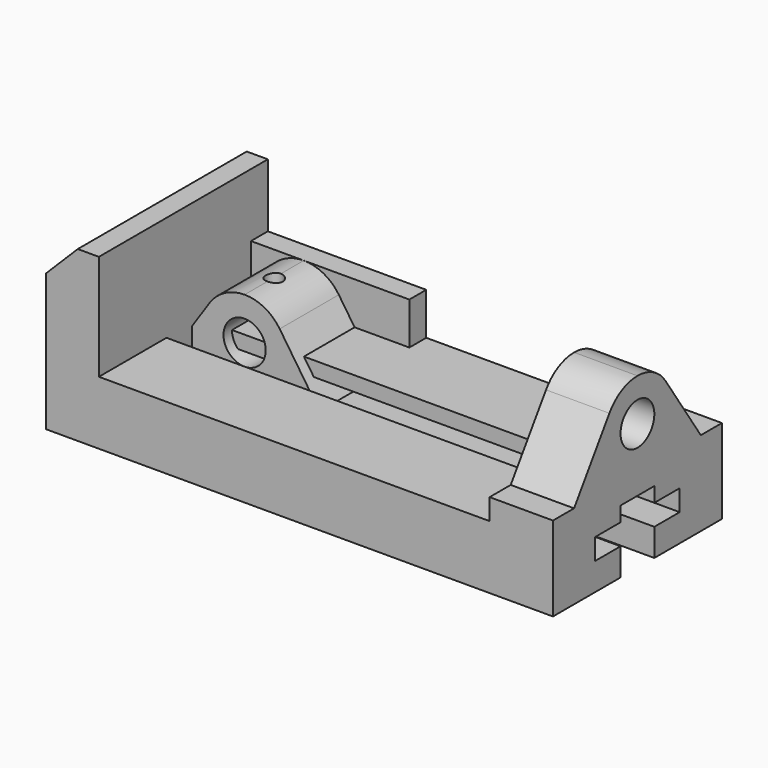
from build123d import *

# Parameters (mm, degrees)
F1_DEPTH  = 127
F2_SIZE2  = 19.05
F2_SIZE   = 19.05
F4_DEPTH  = 273.05
F5_R      = 12.7
F6_DEPTH  = 38.101
F8_DEPTH  = 57.15
F10_DEPTH = 44.45
F9_R      = 12.7
F11_DEPTH = 57.151
F12_R     = 5.08
F13_REACH = 99.4594097937
F14_R     = 12.7
F15_DEPTH = 279.4
F17_DEPTH = 25.4
F18_DEPTH = 2.54
F19_R     = 4.445
F20_DEPTH = 76.2


with BuildPart() as f1:
    # F0 (on Front) → F1 (new body)
    with BuildSketch(Plane.XZ):
        Polygon((31.75, 38.1), (31.75, 101.6), (0, 101.6), (0, 0), (304.8, 0), (304.8, 101.6), (266.7, 101.6), (266.7, 38.1), align=None)
    extrude(amount=F1_DEPTH)

    # F2
    f2_edges = [f1.edges().sort_by_distance(p)[0] for p in [
        (0, -63.5, 101.6),
    ]]
    chamfer(f2_edges, length=F2_SIZE, length2=F2_SIZE2)

    # F3 (on face) → F4 (cut, through all)
    with BuildSketch(Plane.YZ.offset(304.8)):
        Polygon((-76.2, 16.51), (-76.2, 0), (-50.8, 0), (-50.8, 16.51), (-31.75, 16.51), (-31.75, 29.21), (-50.8, 29.21), (-50.8, 38.1), (-76.2, 38.1), (-76.2, 29.21), (-95.25, 29.21), (-95.25, 16.51), align=None)
    extrude(amount=-F4_DEPTH, mode=Mode.SUBTRACT)

    # F5 (on face) → F6 (cut, through all)
    with BuildSketch(Plane(origin=(266.7, 0, 0), x_dir=(0, -1, 0), z_dir=(-1, 0, 0))):
        with BuildLine():
            Line((0, 101.6), (0, 50.8))
            Line((0, 50.8), (15.875, 50.8))
            Line((15.875, 50.8), (42.4065743945, 90.3501730104))
            ThreePointArc((42.4065743945, 90.3501730104), (51.5470588235, 98.6117647059), (63.5, 101.6))
            Line((63.5, 101.6), (0, 101.6))
        make_face()
        with BuildLine():
            Line((84.5934256055, 90.3501730104), (111.125, 50.8))
            Line((111.125, 50.8), (127, 50.8))
            Line((127, 50.8), (127, 101.6))
            Line((127, 101.6), (63.5, 101.6))
            ThreePointArc((63.5, 101.6), (75.4529411765, 98.6117647059), (84.5934256055, 90.3501730104))
        make_face()
        with Locations((63.5, 76.2)):
            Circle(F5_R)
    extrude(amount=-F6_DEPTH, mode=Mode.SUBTRACT)


with BuildPart() as f8:
    # F7 (on Front) → F8 (new body)
    with BuildSketch(Plane.XZ):
        Polygon((0, 63.5), (0, 0), (50.8, 0), (50.8, -8.89), (31.75, -8.89), (31.75, -21.59), (95.25, -21.59), (95.25, -8.89), (76.2, -8.89), (76.2, 0), (127, 0), (127, 63.5), align=None)
    extrude(amount=F8_DEPTH)

    # F9 (on face) → F10 (cut)
    with BuildSketch(Plane.XZ.offset(57.15)):
        with BuildLine():
            Line((0, 63.5), (0, 12.7))
            Line((0, 12.7), (15.875, 12.7))
            Line((15.875, 12.7), (42.4065743945, 52.2501730104))
            ThreePointArc((42.4065743945, 52.2501730104), (51.5470588235, 60.5117647059), (63.5, 63.5))
            Line((63.5, 63.5), (0, 63.5))
        make_face()
        with BuildLine():
            Line((127, 63.5), (63.5, 63.5))
            ThreePointArc((63.5, 63.5), (75.4529411765, 60.5117647059), (84.5934256055, 52.2501730104))
            Line((84.5934256055, 52.2501730104), (111.125, 12.7))
            Line((111.125, 12.7), (127, 12.7))
            Line((127, 12.7), (127, 63.5))
        make_face()
    extrude(amount=-F10_DEPTH, mode=Mode.SUBTRACT)

    # F9 (on face) → F11 (cut, through all)
    with BuildSketch(Plane.XZ.offset(57.15)):
        with Locations((63.5, 38.1)):
            Circle(F9_R)
    extrude(amount=-F11_DEPTH, mode=Mode.SUBTRACT)

    f13_end = f8.faces().sort_by_distance((50.8, -28.575, 38.1))[0]
    # F12 (on face) → F13 (cut, up to a face of the model that its end follows)
    with BuildSketch(Plane.XY.offset(63.5)):
        with Locations((63.5, -34.925)):
            Circle(F12_R)
    f13_long = extrude(amount=-F13_REACH, mode=Mode.PRIVATE)
    add(split(f13_long, bisect_by=f13_end, keep=Keep.ALL, mode=Mode.PRIVATE).solids().sort_by_distance((63.5, -34.925, 63.5))[0], mode=Mode.SUBTRACT)


with BuildPart() as f15:
    # F14 (on Right) → F15 (new body)
    with BuildSketch(Plane.YZ):
        Circle(F14_R)
    extrude(amount=F15_DEPTH)

    # F16 (on face) → F17 (cut)
    with BuildSketch(Plane.YZ.offset(279.4)):
        with BuildLine():
            ThreePointArc((5.8198711326, -2.54), (6.2160550871, -1.2973662374), (6.35, 0))
            ThreePointArc((6.35, 0), (6.2160550871, 1.2973662374), (5.8198711326, 2.54))
            ThreePointArc((5.8198711326, 2.54), (4.4901280605, 4.4901280605), (2.54, 5.8198711326))
            ThreePointArc((2.54, 5.8198711326), (0, 6.35), (-2.54, 5.8198711326))
            ThreePointArc((-2.54, 5.8198711326), (-4.4901280605, 4.4901280605), (-5.8198711326, 2.54))
            ThreePointArc((-5.8198711326, 2.54), (-6.35, 0), (-5.8198711326, -2.54))
            ThreePointArc((-5.8198711326, -2.54), (-4.4901280605, -4.4901280605), (-2.54, -5.8198711326))
            ThreePointArc((-2.54, -5.8198711326), (0, -6.35), (2.54, -5.8198711326))
            ThreePointArc((2.54, -5.8198711326), (4.4901280605, -4.4901280605), (5.8198711326, -2.54))
        make_face()
    extrude(amount=-F17_DEPTH, mode=Mode.SUBTRACT)

    # F16 (on face) → F18 (cut)
    with BuildSketch(Plane.YZ.offset(279.4)):
        with BuildLine():
            ThreePointArc((-5.8198711326, -2.54), (-6.35, 0), (-5.8198711326, 2.54))
            Line((-5.8198711326, 2.54), (-12.4434078933, 2.54))
            ThreePointArc((-12.4434078933, 2.54), (-12.7, 0), (-12.4434078933, -2.54))
            Line((-12.4434078933, -2.54), (-5.8198711326, -2.54))
        make_face()
        with BuildLine():
            ThreePointArc((-2.54, 5.8198711326), (0, 6.35), (2.54, 5.8198711326))
            Line((2.54, 5.8198711326), (2.54, 12.4434078933))
            ThreePointArc((2.54, 12.4434078933), (0, 12.7), (-2.54, 12.4434078933))
            Line((-2.54, 12.4434078933), (-2.54, 5.8198711326))
        make_face()
        with BuildLine():
            ThreePointArc((5.8198711326, 2.54), (6.2160550871, 1.2973662374), (6.35, 0))
            ThreePointArc((6.35, 0), (6.2160550871, -1.2973662374), (5.8198711326, -2.54))
            Line((5.8198711326, -2.54), (12.4434078933, -2.54))
            ThreePointArc((12.4434078933, -2.54), (12.6356891432, -1.2764638175), (12.7, 0))
            ThreePointArc((12.7, 0), (12.6356891432, 1.2764638175), (12.4434078933, 2.54))
            Line((12.4434078933, 2.54), (5.8198711326, 2.54))
        make_face()
        with BuildLine():
            Line((2.54, -12.4434078933), (2.54, -5.8198711326))
            ThreePointArc((2.54, -5.8198711326), (0, -6.35), (-2.54, -5.8198711326))
            Line((-2.54, -5.8198711326), (-2.54, -12.4434078933))
            ThreePointArc((-2.54, -12.4434078933), (0, -12.7), (2.54, -12.4434078933))
        make_face()
    extrude(amount=-F18_DEPTH, mode=Mode.SUBTRACT)


with BuildPart() as f20:
    # F19 (on Right) → F20 (new body, symmetric)
    with BuildSketch(Plane.YZ):
        Circle(F19_R)
    extrude(amount=F20_DEPTH, both=True)

    # F21 (on Front) → F22 (revolve)
    with BuildSketch(Plane.XZ):
        Polygon((0, 15.875), (0, -60.325), (6.35, -60.325), (6.35, -15.875), (15.875, -15.875), (15.875, 15.875), align=None)
    revolve(axis=Axis((0, 0, -22.225), (0, 0, -1)))

    # F23 (on Front) → F24 (revolve)
    with BuildSketch(Plane.XZ):
        with BuildLine():
            Line((-86.36, 0), (-66.04, 0))
            ThreePointArc((-66.04, 0), (-76.2, 10.16), (-86.36, 0))
        make_face()
        with BuildLine():
            Line((66.04, 0), (86.36, 0))
            ThreePointArc((86.36, 0), (76.2, 10.16), (66.04, 0))
        make_face()
    revolve(axis=Axis((-76.2, 0, 0), (1, 0, 0)))


solid = Compound([f1.part, f8.part, f15.part, f20.part])
